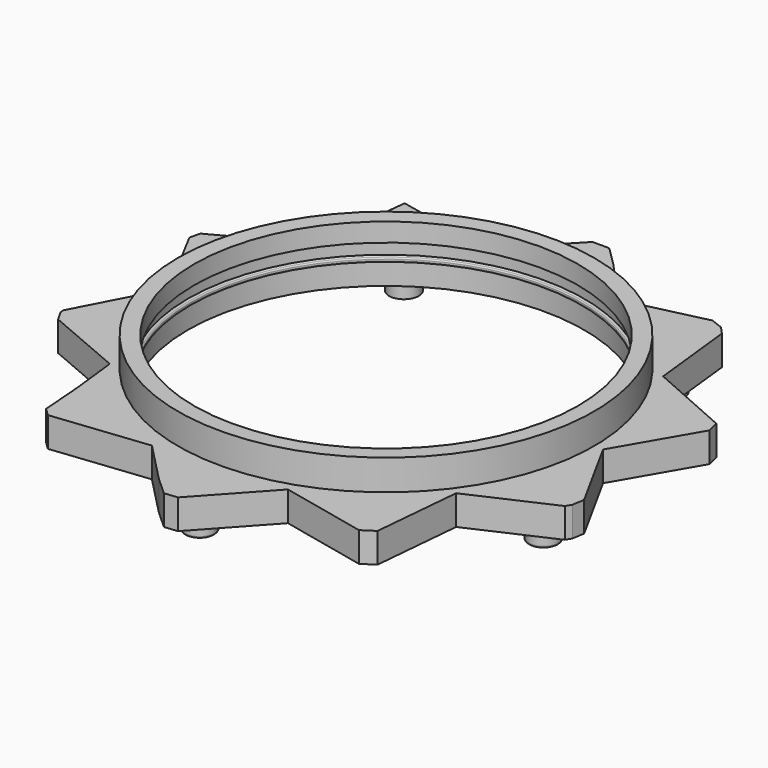
from build123d import *

# Parameters (mm, degrees)
F3_R     = 20.5
F4_DEPTH = 3
F5_R     = 1.5
F6_DEPTH = 2
F7_R     = 0.2
F7_2_R   = 0.2
F7_3_R   = 0.2
F8_R     = 1.5
F9_DEPTH = 2


with BuildPart() as f1:
    # F0 (on Front) → F1 (revolve)
    with BuildSketch(Plane.XZ):
        with BuildLine():
            Line((-21, 4.6640044797), (-21, 1.3408993961))
            Line((-21, 1.3408993961), (-21, 0))
            Line((-21, 0), (-21, -1.4155078679))
            Line((-21, -1.4155078679), (-20, -1.4155078679))
            Line((-20, -1.4155078679), (-20, 0.723031953))
            Line((-20, 0.723031953), (-19.7798779008, 0.8394374288))
            ThreePointArc((-19.7798779008, 0.8394374288), (-19.7215120339, 0.8946373902), (-19.7, 0.9720379235))
            Line((-19.7, 0.9720379235), (-19.7, 1.1202138481))
            ThreePointArc((-19.7, 1.1202138481), (-19.7236004385, 1.2009798734), (-19.7869753447, 1.2563310506))
            Line((-19.7869753447, 1.2563310506), (-20, 1.3549652073))
            Line((-20, 1.3549652073), (-19.9719204218, 2.7546835851))
            Line((-19.9719204218, 2.7546835851), (-19.3768669452, 2.7546835851))
            Line((-19.3768669452, 2.7546835851), (-19.3768669452, 4.6314430072))
            Line((-19.3768669452, 4.6314430072), (-21, 4.6640044797))
        make_face()
        Polygon((-21, -1.4155078679), (-21, 0), (-21.1709106225, 0), (-21.6530393809, 0), (-21.6530393809, -1.4155078679), (-21.2582742561, -1.4155078679), align=None)
    revolve(axis=Axis((0, 0, 4.1345077953), (0, 0, 1)))


with BuildPart() as f4:
    # F3 (on face) → F4 (new body)
    with BuildSketch(Plane(origin=(0, 0, -1.4155078679), x_dir=(1, 0, 0), z_dir=(0, 0, -1))):
        Polygon((-17.0443542302, 17.5880640745), (-17.5802018493, 12.8813311458), (-25.5107674748, 9.4892438501), (-26.1456985027, 8.3832368255), (-26.1456985027, 8.0095588431), (-21.9675619155, 0), (-26.1567309499, -7.8945141286), (-25.8933100849, -8.9481929317), (-23.8518081605, -10.0457752123), (-17.7485514432, -12.7631025389), (-16.5503714234, -23.0435039848), (-6.7929682476, -21.0023011101), (-0.866433722, -27.1395202726), (0.8171786401, -27.1395202726), (2.900598105, -25.0820405781), (6.7568528466, -20.6729657948), (14.8950507864, -22.5767139345), (16.1493904889, -22.0833402127), (16.860185191, -21.30564861), (17.8031453724, -12.707031999), (26.1139851063, -9.0305751648), (26.4153070748, -7.7816629782), (21.907278978, 0), (26.1139851063, 7.6492135413), (25.9108040482, 8.8818427175), (25.5857165903, 9.4236582518), (17.526216805, 13.0673646927), (16.7145878077, 21.9628661871), (15.4829295352, 22.76904881), (6.7750127055, 20.8425968885), (0.8599998546, 27.3143518716), (-0.4512939139, 27.4581538186), (-2.2986123804, 25.7842168212), (-6.2730474904, 21.6959586068), (-15.9318167716, 22.7551795542), (-16.7042777427, 22.0092364009), align=None)
        Circle(F3_R, mode=Mode.SUBTRACT)
    extrude(amount=-F4_DEPTH)


with BuildPart() as f6:
    # F5 (on face) → F6 (new body)
    with BuildSketch(Plane(origin=(0, 0, -1.4155078679), x_dir=(1, 0, 0), z_dir=(0, 0, -1))):
        with Locations((21.8569319695, 7.4604498222)):
            Circle(F5_R)
    extrude(amount=F6_DEPTH)

    # F7
    f7_edges = [f6.edges().sort_by_distance(p)[0] for p in [
        (20.356932, -7.46045, -3.415508),
    ]]
    fillet(f7_edges, radius=F7_R)


with BuildPart() as f6b:
    # F5 (on face) → F6, piece 2 (new body)
    with BuildSketch(Plane(origin=(0, 0, -1.4155078679), x_dir=(1, 0, 0), z_dir=(0, 0, -1))):
        with Locations((-0.3411459945, 23.0925833566)):
            Circle(F5_R)
    extrude(amount=F6_DEPTH)

    # F7#2
    f7_2_edges = [f6b.edges().sort_by_distance(p)[0] for p in [
        (-1.841146, -23.092583, -3.415508),
    ]]
    fillet(f7_2_edges, radius=F7_2_R)


with BuildPart() as f6c:
    # F5 (on face) → F6, piece 3 (new body)
    with BuildSketch(Plane(origin=(0, 0, -1.4155078679), x_dir=(1, 0, 0), z_dir=(0, 0, -1))):
        with Locations((-22.0677717892, 6.8115515802)):
            Circle(F5_R)
    extrude(amount=F6_DEPTH)

    # F7#3
    f7_3_edges = [f6c.edges().sort_by_distance(p)[0] for p in [
        (-23.567772, -6.811552, -3.415508),
    ]]
    fillet(f7_3_edges, radius=F7_3_R)


with BuildPart() as f6d:
    # F5 (on face) → F6, piece 4 (new body)
    with BuildSketch(Plane(origin=(0, 0, -1.4155078679), x_dir=(1, 0, 0), z_dir=(0, 0, -1))):
        with Locations((-13.2974870273, -18.8828129639)):
            Circle(F5_R)
    extrude(amount=F6_DEPTH)


with BuildPart() as f6e:
    # F5 (on face) → F6, piece 5 (new body)
    with BuildSketch(Plane(origin=(0, 0, -1.4155078679), x_dir=(1, 0, 0), z_dir=(0, 0, -1))):
        with Locations((13.8494728414, -18.4817717951)):
            Circle(F5_R)
    extrude(amount=F6_DEPTH)


with BuildPart() as f9:
    # F8 (on offset) → F9 (new body)
    with BuildSketch(Plane.XY.offset(-1.56)):
        with Locations((13.2974870273, -18.8828129639)):
            Circle(F8_R)
    extrude(amount=F9_DEPTH)


with BuildPart() as f9b:
    # F8 (on offset) → F9, piece 2 (new body)
    with BuildSketch(Plane.XY.offset(-1.56)):
        with Locations((22.0677717892, 6.8115515802)):
            Circle(F8_R)
    extrude(amount=F9_DEPTH)


with BuildPart() as f9c:
    # F8 (on offset) → F9, piece 3 (new body)
    with BuildSketch(Plane.XY.offset(-1.56)):
        with Locations((0.3411459945, 23.0925833566)):
            Circle(F8_R)
    extrude(amount=F9_DEPTH)


with BuildPart() as f9d:
    # F8 (on offset) → F9, piece 4 (new body)
    with BuildSketch(Plane.XY.offset(-1.56)):
        with Locations((-21.8569319695, 7.4604498222)):
            Circle(F8_R)
    extrude(amount=F9_DEPTH)


with BuildPart() as f9e:
    # F8 (on offset) → F9, piece 5 (new body)
    with BuildSketch(Plane.XY.offset(-1.56)):
        with Locations((-13.8494728414, -18.4817717951)):
            Circle(F8_R)
    extrude(amount=F9_DEPTH)


solid = Compound([f1.part, f4.part, f6.part, f6b.part, f6c.part, f6d.part, f6e.part, f9.part, f9b.part, f9c.part, f9d.part, f9e.part])
